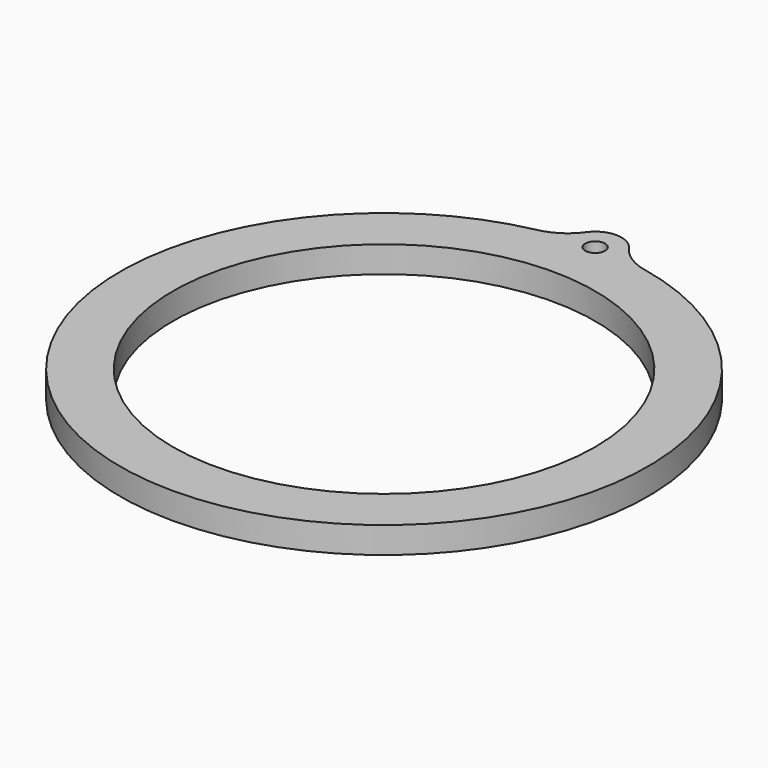
from build123d import *

# Parameters (mm, degrees)
F0_R     = 20.32
F0_R_2   = 0.9525
F1_DEPTH = 2.54
F2_R     = 5.08


with BuildPart() as f1:
    # F0 (on Top) → F1 (new body)
    with BuildSketch(Plane.XY):
        with BuildLine():
            ThreePointArc((2.5368230131, 25.273), (0, 27.94), (-2.5368230131, 25.273))
            ThreePointArc((-2.5368230131, 25.273), (0, -25.4), (2.5368230131, 25.273))
        make_face()
        Circle(F0_R, mode=Mode.SUBTRACT)
        with Locations((0, 25.4)):
            Circle(F0_R_2, mode=Mode.SUBTRACT)
    extrude(amount=F1_DEPTH)

    # F2
    f2_edges = [f1.edges().sort_by_distance(p)[0] for p in [
        (-2.536823, 25.273, 1.27),
        (2.536823, 25.273, 1.27),
    ]]
    fillet(f2_edges, radius=F2_R)


solid = f1.part
